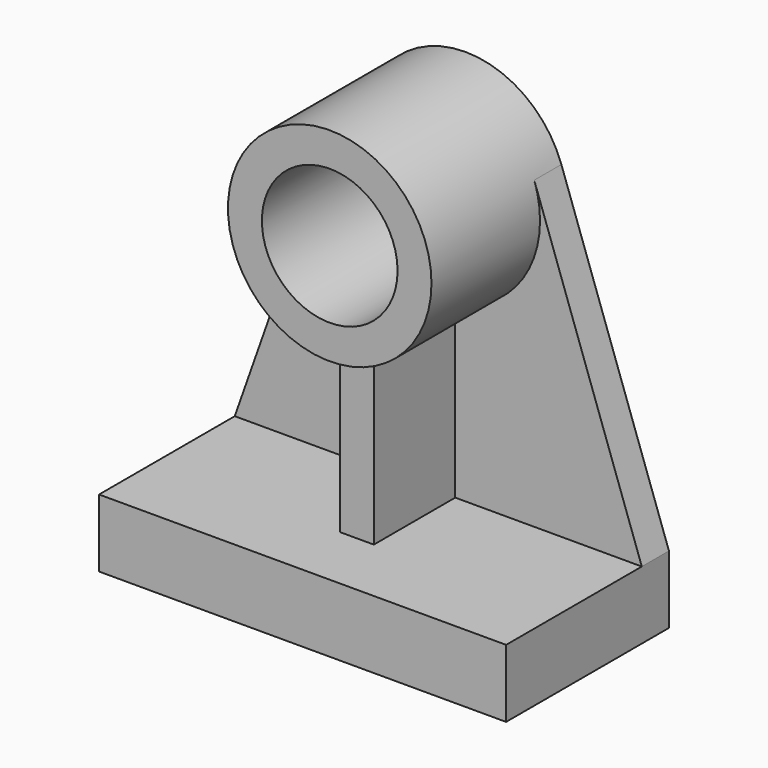
from build123d import *

# Parameters (mm, degrees)
F0_R     = 76.2
F0_R_2   = 50.8
F1_DEPTH = 127
F3_DEPTH = 25.4
F4_W     = 304.8
F4_H     = 50.8
F5_DEPTH = 152.4
F7_DEPTH = 76.2


with BuildPart() as f1:
    # F0 (on Front) → F1 (new body)
    with BuildSketch(Plane.XZ):
        Circle(F0_R)
        Circle(F0_R_2, mode=Mode.SUBTRACT)
    extrude(amount=F1_DEPTH)

    # F2 (on Front) → F3 (join)
    with BuildSketch(Plane.XZ):
        with BuildLine():
            ThreePointArc((0, -76.2), (-62.1944082776, -44.0260783968), (-71.8681337184, 25.3261002888))
            Line((-71.8681337184, 25.3261002888), (-152.4, -203.2))
            Line((-152.4, -203.2), (0, -203.2))
            Line((0, -203.2), (0, -76.2))
        make_face()
        with BuildLine():
            ThreePointArc((71.8681337184, 25.3261002888), (62.1944082776, -44.0260783968), (0, -76.2))
            Line((0, -76.2), (0, -203.2))
            Line((0, -203.2), (152.4, -203.2))
            Line((152.4, -203.2), (71.8681337184, 25.3261002888))
        make_face()
    extrude(amount=F3_DEPTH)

    # F4 (on face) → F5 (join)
    with BuildSketch(Plane(origin=(0, 0, 0), x_dir=(-1, 0, 0), z_dir=(0, 1, 0))):
        with Locations((0, -228.6)):
            Rectangle(F4_W, F4_H)
    extrude(amount=-F5_DEPTH)

    # F6 (on face) → F7 (join)
    with BuildSketch(Plane.XZ.offset(25.4)):
        with BuildLine():
            Line((0, -203.2), (0, -76.2))
            ThreePointArc((0, -76.2), (-6.3723210333, -75.9330858365), (-12.7, -75.1342132454))
            Line((-12.7, -75.1342132454), (-12.7, -203.2))
            Line((-12.7, -203.2), (0, -203.2))
        make_face()
        with BuildLine():
            ThreePointArc((12.7, -75.1342132454), (6.3723210333, -75.9330858365), (0, -76.2))
            Line((0, -76.2), (0, -203.2))
            Line((0, -203.2), (12.7, -203.2))
            Line((12.7, -203.2), (12.7, -75.1342132454))
        make_face()
    extrude(amount=F7_DEPTH)


solid = f1.part
